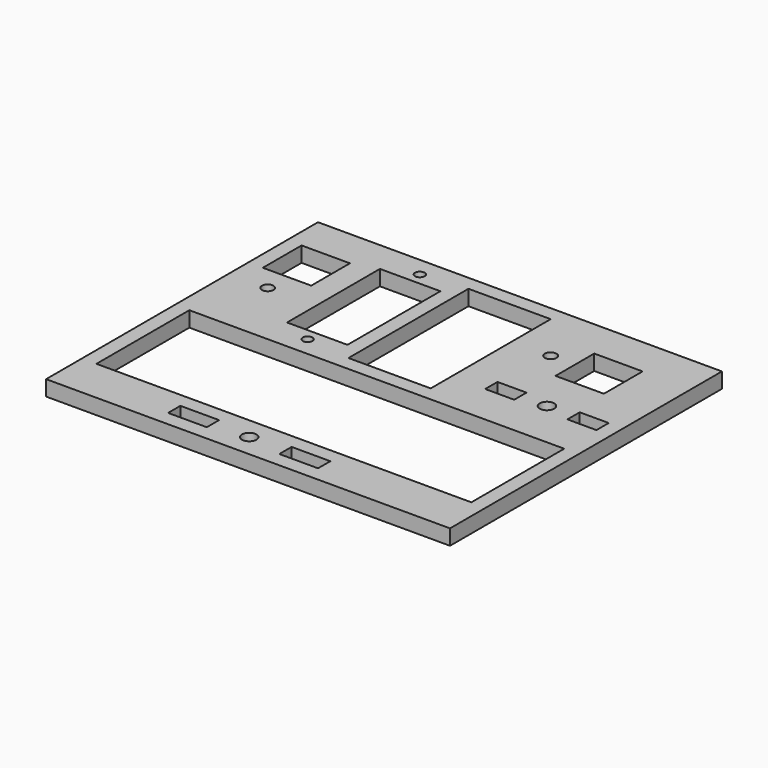
from build123d import *

# Parameters (mm, degrees)
F0_W     = 83.5
F0_H     = 70.2625
F0_W_2   = 8
F0_H_2   = 3.175
F0_W_3   = 77.5
F0_H_3   = 24
F0_R     = 1
F0_W_4   = 6
F0_W_5   = 17
F0_H_4   = 31
F0_W_6   = 10
F0_H_5   = 10
F0_R_2   = 1.2
F1_DEPTH = 3.175


# Not quite as in the source:
# - a length typed as a fraction of an inch, garbled in the dataset ("3 / 203.2 mm" for 3/8 in), is restored
# - a feature names something its author has since deleted; it is built from what else it names


with BuildPart() as f1:
    # F0 (on Top) → F1 (new body)
    with BuildSketch(Plane.XY):
        with Locations((2.5199788651, 27.2772044539)):
            Rectangle(F0_W, F0_H)
        with Locations((-12.4800211349, -3.1790455461)):
            Rectangle(F0_W_2, F0_H_2, mode=Mode.SUBTRACT)
        with BuildLine():
            ThreePointArc((-0.9800211349, -4.6790455461), (-2.0406813067, -2.1183853743), (0.5199788651, -3.1790455461))
            ThreePointArc((0.5199788651, -3.1790455461), (0.0806390368, -4.2397057179), (-0.9800211349, -4.6790455461))
        make_face(mode=Mode.SUBTRACT)
        with Locations((10.5199788651, -3.1790455461)):
            Rectangle(F0_W_2, F0_H_2, mode=Mode.SUBTRACT)
        with Locations((2.5199788651, 13.4084544539)):
            Rectangle(F0_W_3, F0_H_3, mode=Mode.SUBTRACT)
        Polygon((-36.2300211349, 34.4084544539), (-36.230021135, 44.4084544539), (-36.230021135, 54.4084544539), (-26.230021135, 54.4084544539), (-26.230021135, 44.4084544539), (-26.2300211349, 34.4084544539), align=None, mode=Mode.SUBTRACT)
        with Locations((-14.980021135, 29.4084544539)):
            Circle(F0_R, mode=Mode.SUBTRACT)
        Polygon((-21.230021135, 31.9084544539), (-21.230021135, 55.9084544539), (-8.730021135, 55.9084544539), (-8.730021135, 43.9084544539), (-8.730021135, 31.9084544539), align=None, mode=Mode.SUBTRACT)
        with Locations((-14.980021135, 58.4084544539)):
            Circle(F0_R, mode=Mode.SUBTRACT)
        with Locations((21.2699788651, 35.3209544539)):
            Rectangle(F0_W_4, F0_H_2, mode=Mode.SUBTRACT)
        with Locations((2.7699788651, 43.9084544539)):
            Rectangle(F0_W_5, F0_H_4, mode=Mode.SUBTRACT)
        with BuildLine():
            ThreePointArc((29.7699788651, 33.8209544539), (28.7093186933, 36.3816146257), (31.2699788651, 35.3209544539))
            ThreePointArc((31.2699788651, 35.3209544539), (30.8306390368, 34.2602942821), (29.7699788651, 33.8209544539))
        make_face(mode=Mode.SUBTRACT)
        with Locations((38.2699788651, 35.3209544539)):
            Rectangle(F0_W_4, F0_H_2, mode=Mode.SUBTRACT)
        Polygon((14.2699788651, 54.4084544539), (24.2699788651, 54.4084544539), (34.2699788651, 54.4084544539), (34.2699788651, 44.4084544539), (24.2699788651, 44.4084544539), (14.2699788651, 44.4084544539), align=None, mode=Mode.SUBTRACT)
        with Locations((-31.2300211349, 39.4084544539)):
            Rectangle(F0_W_6, F0_H_5)
        with Locations((-31.230021135, 39.4084544539)):
            Circle(F0_R_2, mode=Mode.SUBTRACT)
        with Locations((19.2699788651, 49.4084544539)):
            Rectangle(F0_W_6, F0_H_5)
        with Locations((19.2699788651, 49.4084544539)):
            Circle(F0_R_2, mode=Mode.SUBTRACT)
    extrude(amount=F1_DEPTH)


solid = f1.part
